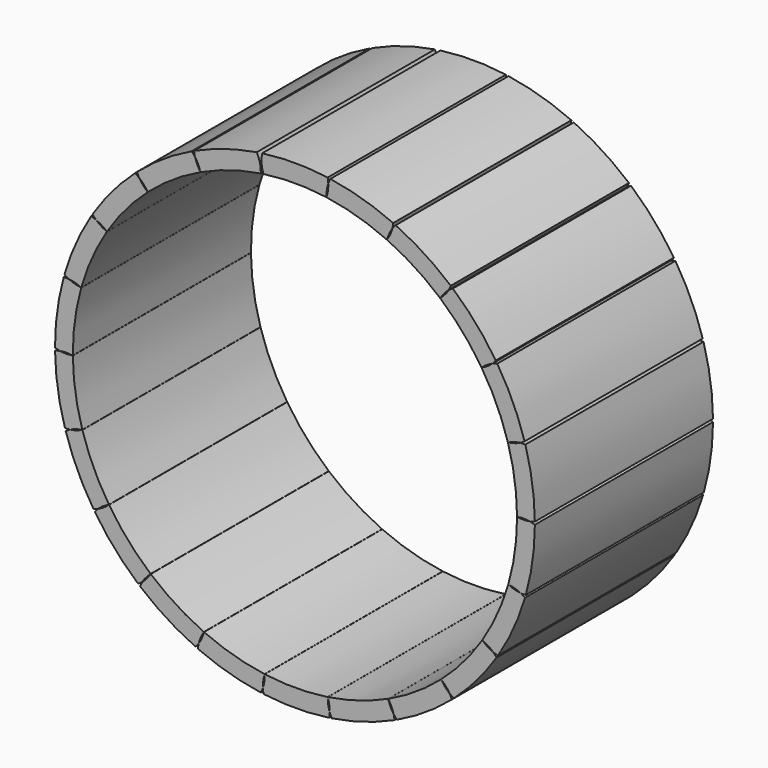
from build123d import *

# Parameters (mm, degrees)
F1_DEPTH      = 5
F1_DEPTH_BACK = 5


with BuildPart() as f1:
    # F0 (on Front) → F1 (new body, two sides)
    with BuildSketch(Plane.XZ) as f1_sk:
        with BuildLine():
            ThreePointArc((1.4985057046, 10.441937681), (1.4996263796, 10.408477179), (1.5, 10.375))
            ThreePointArc((1.5, 10.375), (1.4796631944, 10.1288357639), (1.4192042252, 9.8893464534))
            ThreePointArc((1.4192042252, 9.8893464534), (1.4195814524, 9.8813770901), (1.4200010621, 9.8734098458))
            ThreePointArc((1.4200010621, 9.8734098458), (2.8052199084, 9.5724273967), (4.1337871536, 9.0781291448))
            ThreePointArc((4.1337871536, 9.0781291448), (4.1384407168, 9.084609685), (4.1430597453, 9.0911148852))
            ThreePointArc((4.1430597453, 9.0911148852), (4.2349711699, 9.3559736019), (4.3745632608, 9.5991029871))
            ThreePointArc((4.3745632608, 9.5991029871), (4.3979930653, 9.7138757212), (4.4123952899, 9.830126795))
            ThreePointArc((4.4123952899, 9.830126795), (3.0301999512, 10.3401408721), (1.5913530114, 10.6568391464))
            ThreePointArc((1.5913530114, 10.6568391464), (1.5407305697, 10.5512024832), (1.4985057046, 10.441937681))
        make_face()
    extrude(amount=F1_DEPTH)
    extrude(f1_sk.sketch, amount=-F1_DEPTH_BACK)


with BuildPart() as f1b:
    # F0 (on Front) → F1, piece 2 (new body, two sides)
    with BuildSketch(Plane.XZ) as f1_2_sk:
        with BuildLine():
            ThreePointArc((1.4192042252, 9.8893464534), (1.4329213675, 10.1693637561), (1.4985057046, 10.441937681))
            ThreePointArc((1.4985057046, 10.441937681), (1.4887129572, 10.5586674472), (1.4698412201, 10.6742771084))
            ThreePointArc((1.4698412201, 10.6742771084), (0, 10.775), (-1.4698412201, 10.6742771084))
            ThreePointArc((-1.4698412201, 10.6742771084), (-1.496353621, 10.2704732533), (-1.4139577737, 9.8742771084))
            ThreePointArc((-1.4139577737, 9.8742771084), (0, 9.975), (1.4139577737, 9.8742771084))
            ThreePointArc((1.4139577737, 9.8742771084), (1.4166010374, 9.8818048046), (1.4192042252, 9.8893464534))
        make_face()
    extrude(amount=F1_DEPTH)
    extrude(f1_2_sk.sketch, amount=-F1_DEPTH_BACK)


with BuildPart() as f1c:
    # F0 (on Front) → F1, piece 3 (new body, two sides)
    with BuildSketch(Plane.XZ) as f1_3_sk:
        with BuildLine():
            ThreePointArc((-1.5333564365, 9.9216618431), (-1.5795383622, 10.2910031579), (-1.7152404456, 10.6376019485))
            ThreePointArc((-1.7152404456, 10.6376019485), (-3.1503051184, 10.3041837455), (-4.5264727442, 9.7781219821))
            ThreePointArc((-4.5264727442, 9.7781219821), (-4.5107188823, 9.6620463513), (-4.4859552526, 9.5475539984))
            ThreePointArc((-4.4859552526, 9.5475539984), (-4.343543736, 9.3060652622), (-4.2485568314, 9.0422938881))
            ThreePointArc((-4.2485568314, 9.0422938881), (-4.2438624259, 9.0358428719), (-4.2391337748, 9.0294169158))
            ThreePointArc((-4.2391337748, 9.0294169158), (-2.9164077546, 9.5391399407), (-1.5347846874, 9.8562194052))
            ThreePointArc((-1.5347846874, 9.8562194052), (-1.5337135417, 9.8889328324), (-1.5333564365, 9.9216618431))
        make_face()
    extrude(amount=F1_DEPTH)
    extrude(f1_3_sk.sketch, amount=-F1_DEPTH_BACK)


with BuildPart() as f1d:
    # F0 (on Front) → F1, piece 4 (new body, two sides)
    with BuildSketch(Plane.XZ) as f1_4_sk:
        with BuildLine():
            ThreePointArc((4.5240990976, 9.779220437), (4.445812008, 9.6920833735), (4.3745632608, 9.5991029871))
            ThreePointArc((4.3745632608, 9.5991029871), (4.2826518361, 9.3342442704), (4.1430597453, 9.0911148852))
            ThreePointArc((4.1430597453, 9.0911148852), (4.1411805637, 9.0833610649), (4.13934265, 9.0755973592))
            ThreePointArc((4.13934265, 9.0755973592), (5.3840128131, 8.3972037625), (6.5199524821, 7.5492280818))
            ThreePointArc((6.5199524821, 7.5492280818), (6.5262407264, 7.5541383809), (6.5325027647, 7.5590820566))
            ThreePointArc((6.5325027647, 7.5590820566), (6.6951897205, 7.7874037687), (6.8975222064, 7.9814641071))
            ThreePointArc((6.8975222064, 7.9814641071), (6.9522833955, 8.0850157773), (6.9987970873, 8.1925249057))
            ThreePointArc((6.9987970873, 8.1925249057), (5.8158133394, 9.0706637134), (4.5240990976, 9.779220437))
        make_face()
    extrude(amount=F1_DEPTH)
    extrude(f1_4_sk.sketch, amount=-F1_DEPTH_BACK)


with BuildPart() as f1e:
    # F0 (on Front) → F1, piece 5 (new body, two sides)
    with BuildSketch(Plane.XZ) as f1_5_sk:
        with BuildLine():
            ThreePointArc((-4.2485568314, 9.0422938881), (-4.390968348, 9.2837826244), (-4.4859552526, 9.5475539984))
            ThreePointArc((-4.4859552526, 9.5475539984), (-4.5582810283, 9.6396990926), (-4.6375766814, 9.7259193665))
            ThreePointArc((-4.6375766814, 9.7259193665), (-5.9209592387, 9.002381168), (-7.0936455296, 8.1105374729))
            ThreePointArc((-7.0936455296, 8.1105374729), (-7.0458840891, 8.0035768212), (-6.9899217557, 7.9006693216))
            ThreePointArc((-6.9899217557, 7.9006693216), (-6.7853450225, 7.7089763118), (-6.6200124954, 7.4825629612))
            ThreePointArc((-6.6200124954, 7.4825629612), (-6.6136933601, 7.4776924806), (-6.6073484088, 7.4728556793))
            ThreePointArc((-6.6073484088, 7.4728556793), (-5.4813520563, 8.3339909188), (-4.2446594372, 9.0268206619))
            ThreePointArc((-4.2446594372, 9.0268206619), (-4.2465875593, 9.0345624574), (-4.2485568314, 9.0422938881))
        make_face()
    extrude(amount=F1_DEPTH)
    extrude(f1_5_sk.sketch, amount=-F1_DEPTH_BACK)


with BuildPart() as f1f:
    # F0 (on Front) → F1, piece 6 (new body, two sides)
    with BuildSketch(Plane.XZ) as f1_6_sk:
        with BuildLine():
            ThreePointArc((7.091676592, 8.1122591252), (6.9920438997, 8.0506550438), (6.8975222064, 7.9814641071))
            ThreePointArc((6.8975222064, 7.9814641071), (6.7348352505, 7.753142395), (6.5325027647, 7.5590820566))
            ThreePointArc((6.5325027647, 7.5590820566), (6.5285188549, 7.5521696391), (6.5245717674, 7.5452361296))
            ThreePointArc((6.5245717674, 7.5452361296), (7.5282280627, 6.5441888142), (8.3798512956, 5.4109811739))
            ThreePointArc((8.3798512956, 5.4109811739), (8.387266657, 5.4139248905), (8.3946662565, 5.4169080066))
            ThreePointArc((8.3946662565, 5.4169080066), (8.6149972525, 5.5902634276), (8.8637386015, 5.7195908845))
            ThreePointArc((8.8637386015, 5.7195908845), (8.9454110539, 5.8035631819), (9.0202817993, 5.8936526247))
            ThreePointArc((9.0202817993, 5.8936526247), (8.1319957269, 7.0690360374), (7.091676592, 8.1122591252))
        make_face()
    extrude(amount=F1_DEPTH)
    extrude(f1_6_sk.sketch, amount=-F1_DEPTH_BACK)


with BuildPart() as f1g:
    # F0 (on Front) → F1, piece 7 (new body, two sides)
    with BuildSketch(Plane.XZ) as f1_7_sk:
        with BuildLine():
            ThreePointArc((-6.6200124954, 7.4825629612), (-6.8245892287, 7.6742559711), (-6.9899217557, 7.9006693216))
            ThreePointArc((-6.9899217557, 7.9006693216), (-7.0852421056, 7.9687557896), (-7.1855848335, 8.029196448))
            ThreePointArc((-7.1855848335, 8.029196448), (-8.2136953691, 6.9739395884), (-9.0882454133, 5.7883002953))
            ThreePointArc((-9.0882454133, 5.7883002953), (-9.0123315214, 5.6990880918), (-8.9296875575, 5.6160717593))
            ThreePointArc((-8.9296875575, 5.6160717593), (-8.679458287, 5.4896472285), (-8.4571251692, 5.318867152))
            ThreePointArc((-8.4571251692, 5.318867152), (-8.4496913613, 5.3159703342), (-8.4422422509, 5.3131130966))
            ThreePointArc((-8.4422422509, 5.3131130966), (-7.6038618382, 6.4561528905), (-6.6119209341, 7.4688102507))
            ThreePointArc((-6.6119209341, 7.4688102507), (-6.6159484275, 7.4756973655), (-6.6200124954, 7.4825629612))
        make_face()
    extrude(amount=F1_DEPTH)
    extrude(f1_7_sk.sketch, amount=-F1_DEPTH_BACK)


with BuildPart() as f1h:
    # F0 (on Front) → F1, piece 8 (new body, two sides)
    with BuildSketch(Plane.XZ) as f1_8_sk:
        with BuildLine():
            ThreePointArc((9.0868401101, 5.7905061793), (8.9739037984, 5.7594075343), (8.8637386015, 5.7195908845))
            ThreePointArc((8.8637386015, 5.7195908845), (8.6434076054, 5.5462354635), (8.3946662565, 5.4169080066))
            ThreePointArc((8.3946662565, 5.4169080066), (8.3888991849, 5.4113949367), (8.3831615181, 5.4058512707))
            ThreePointArc((8.3831615181, 5.4058512707), (9.0647925115, 4.1629510835), (9.5633594221, 2.8359798244))
            ThreePointArc((9.5633594221, 2.8359798244), (9.5713033601, 2.8367193526), (9.5792432523, 2.8375011229))
            ThreePointArc((9.5792432523, 2.8375011229), (9.8394339832, 2.9418976426), (10.1145067111, 2.9960533827))
            ThreePointArc((10.1145067111, 2.9960533827), (10.2164981278, 3.0536683733), (10.3136826364, 3.1190664429))
            ThreePointArc((10.3136826364, 3.1190664429), (9.7917934147, 4.496821847), (9.0868401101, 5.7905061793))
        make_face()
    extrude(amount=F1_DEPTH)
    extrude(f1_8_sk.sketch, amount=-F1_DEPTH_BACK)


with BuildPart() as f1i:
    # F0 (on Front) → F1, piece 9 (new body, two sides)
    with BuildSketch(Plane.XZ) as f1_9_sk:
        with BuildLine():
            ThreePointArc((-8.4571251692, 5.318867152), (-8.7073544397, 5.4452916828), (-8.9296875575, 5.6160717593))
            ThreePointArc((-8.9296875575, 5.6160717593), (-9.0403085745, 5.6546039126), (-9.1535990823, 5.6843864084))
            ThreePointArc((-9.1535990823, 5.6843864084), (-9.8434523061, 4.3825873291), (-10.3492756498, 2.9988528682))
            ThreePointArc((-10.3492756498, 2.9988528682), (-10.2513367959, 2.9345899931), (-10.1486819174, 2.8781655998))
            ThreePointArc((-10.1486819174, 2.8781655998), (-9.8729976933, 2.82721407), (-9.611609894, 2.7258520053))
            ThreePointArc((-9.611609894, 2.7258520053), (-9.6036614431, 2.7251626707), (-9.5957094382, 2.7245156224))
            ThreePointArc((-9.5957094382, 2.7245156224), (-9.11261594, 4.0571980147), (-8.4454925616, 5.3079450254))
            ThreePointArc((-8.4454925616, 5.3079450254), (-8.451294342, 5.3134215568), (-8.4571251692, 5.318867152))
        make_face()
    extrude(amount=F1_DEPTH)
    extrude(f1_9_sk.sketch, amount=-F1_DEPTH_BACK)


with BuildPart() as f1j:
    # F0 (on Front) → F1, piece 10 (new body, two sides)
    with BuildSketch(Plane.XZ) as f1_10_sk:
        with BuildLine():
            ThreePointArc((10.3485474119, 3.0013649334), (10.2314232833, 3.0032818926), (10.1145067111, 2.9960533827))
            ThreePointArc((10.1145067111, 2.9960533827), (9.8543159802, 2.8916568629), (9.5792432523, 2.8375011229))
            ThreePointArc((9.5792432523, 2.8375011229), (9.5721585158, 2.8338323953), (9.5650933928, 2.8301260372))
            ThreePointArc((9.5650933928, 2.8301260372), (9.8696803448, 1.4456952966), (9.9749484511, 0.0320686441))
            ThreePointArc((9.9749484511, 0.0320686441), (9.9827797603, 0.030544292), (9.9906190665, 0.0290616148))
            ThreePointArc((9.9906190665, 0.0290616148), (10.2696678962, 0.0560727313), (10.548869147, 0.030685503))
            ThreePointArc((10.548869147, 0.030685503), (10.6629471571, 0.0572927172), (10.7746010538, 0.0927207228))
            ThreePointArc((10.7746010538, 0.0927207228), (10.6612336557, 1.561640784), (10.3485474119, 3.0013649334))
        make_face()
    extrude(amount=F1_DEPTH)
    extrude(f1_10_sk.sketch, amount=-F1_DEPTH_BACK)


with BuildPart() as f1k:
    # F0 (on Front) → F1, piece 11 (new body, two sides)
    with BuildSketch(Plane.XZ) as f1_11_sk:
        with BuildLine():
            ThreePointArc((-9.611609894, 2.7258520053), (-9.887294118, 2.7768035352), (-10.1486819174, 2.8781655998))
            ThreePointArc((-10.1486819174, 2.8781655998), (-10.265674681, 2.8840332651), (-10.3827685769, 2.8807536652))
            ThreePointArc((-10.3827685769, 2.8807536652), (-10.6786820811, 1.4374887861), (-10.7749505298, -0.0326509008))
            ThreePointArc((-10.7749505298, -0.0326509008), (-10.6628919769, -0.0667773854), (-10.548512107, -0.0920554705))
            ThreePointArc((-10.548512107, -0.0920554705), (-10.269625143, -0.06342138), (-9.9902809211, -0.0871838608))
            ThreePointArc((-9.9902809211, -0.0871838608), (-9.9824593969, -0.0856100716), (-9.9746463541, -0.0839947032))
            ThreePointArc((-9.9746463541, -0.0839947032), (-9.8858332955, 1.3307610804), (-9.5973751813, 2.7186420562))
            ThreePointArc((-9.5973751813, 2.7186420562), (-9.6044829504, 2.7222659589), (-9.611609894, 2.7258520053))
        make_face()
    extrude(amount=F1_DEPTH)
    extrude(f1_11_sk.sketch, amount=-F1_DEPTH_BACK)


with BuildPart() as f1l:
    # F0 (on Front) → F1, piece 12 (new body, two sides)
    with BuildSketch(Plane.XZ) as f1_12_sk:
        with BuildLine():
            ThreePointArc((10.7749581379, -0.0300354193), (10.6631000201, 0.0047424144), (10.548869147, 0.030685503))
            ThreePointArc((10.548869147, 0.030685503), (10.2698203173, 0.0036743865), (9.9906190665, 0.0290616148))
            ThreePointArc((9.9906190665, 0.0290616148), (9.9827885188, 0.0275333558), (9.9749662104, 0.0259634689))
            ThreePointArc((9.9749662104, 0.0259634689), (9.9749915526, 0.0129817455), (9.975, 0))
            ThreePointArc((9.975, 0), (9.8761089107, -1.4011059144), (9.5813964344, -2.7744309988))
            ThreePointArc((9.5813964344, -2.7744309988), (9.5884830004, -2.7780961913), (9.5955889607, -2.7817236396))
            ThreePointArc((9.5955889607, -2.7817236396), (9.870972097, -2.834278164), (10.1317657755, -2.9371591972))
            ThreePointArc((10.1317657755, -2.9371591972), (10.2487224227, -2.9437073956), (10.3658334169, -2.9411090721))
            ThreePointArc((10.3658334169, -2.9411090721), (10.6701384407, -1.4995901628), (10.7749581379, -0.0300354193))
        make_face()
    extrude(amount=F1_DEPTH)
    extrude(f1_12_sk.sketch, amount=-F1_DEPTH_BACK)


with BuildPart() as f1m:
    # F0 (on Front) → F1, piece 13 (new body, two sides)
    with BuildSketch(Plane.XZ) as f1_13_sk:
        with BuildLine():
            ThreePointArc((-9.9902809211, -0.0871838608), (-10.2691678851, -0.1158179513), (-10.548512107, -0.0920554705))
            ThreePointArc((-10.548512107, -0.0920554705), (-10.6624333929, -0.1193259097), (-10.7738792894, -0.1554028881))
            ThreePointArc((-10.7738792894, -0.1554028881), (-10.6519680276, -1.6236385495), (-10.3309111471, -3.0615192096))
            ThreePointArc((-10.3309111471, -3.0615192096), (-10.2137778483, -3.0627547397), (-10.0969053081, -3.0548461629))
            ThreePointArc((-10.0969053081, -3.0548461629), (-9.8373263314, -2.9489376901), (-9.5625733222, -2.8931825672))
            ThreePointArc((-9.5625733222, -2.8931825672), (-9.5555100492, -2.8894726847), (-9.5484666084, -2.8857252863))
            ThreePointArc((-9.5484666084, -2.8857252863), (-9.861102652, -1.5030899797), (-9.9745930769, -0.0900996718))
            ThreePointArc((-9.9745930769, -0.0900996718), (-9.9824331218, -0.0886209059), (-9.9902809211, -0.0871838608))
        make_face()
    extrude(amount=F1_DEPTH)
    extrude(f1_13_sk.sketch, amount=-F1_DEPTH_BACK)


with BuildPart() as f1n:
    # F0 (on Front) → F1, piece 14 (new body, two sides)
    with BuildSketch(Plane.XZ) as f1_14_sk:
        with BuildLine():
            ThreePointArc((10.1317657755, -2.9371591972), (9.8563826392, -2.8846046729), (9.5955889607, -2.7817236396))
            ThreePointArc((9.5955889607, -2.7817236396), (9.5876446547, -2.7809880747), (9.5796965487, -2.7802947747))
            ThreePointArc((9.5796965487, -2.7802947747), (9.0888580378, -4.1101441056), (8.4144694391, -5.3569888051))
            ThreePointArc((8.4144694391, -5.3569888051), (8.4202392604, -5.3624989971), (8.4260383079, -5.3679784224))
            ThreePointArc((8.4260383079, -5.3679784224), (8.6755278398, -5.4958565803), (8.8968636424, -5.667927241))
            ThreePointArc((8.8968636424, -5.667927241), (9.0072586175, -5.7071023056), (9.1203739416, -5.7375433912))
            ThreePointArc((9.1203739416, -5.7375433912), (9.8177890082, -4.4397797231), (10.3316539871, -3.0590114237))
            ThreePointArc((10.3316539871, -3.0590114237), (10.2340906548, -2.9941798541), (10.1317657755, -2.9371591972))
        make_face()
    extrude(amount=F1_DEPTH)
    extrude(f1_14_sk.sketch, amount=-F1_DEPTH_BACK)


with BuildPart() as f1o:
    # F0 (on Front) → F1, piece 15 (new body, two sides)
    with BuildSketch(Plane.XZ) as f1_15_sk:
        with BuildLine():
            ThreePointArc((-9.5625733222, -2.8931825672), (-9.8221522989, -2.9990910401), (-10.0969053081, -3.0548461629))
            ThreePointArc((-10.0969053081, -3.0548461629), (-10.1985598103, -3.1130535371), (-10.2953622058, -3.1790158934))
            ThreePointArc((-10.2953622058, -3.1790158934), (-9.7654664053, -4.5537117703), (-9.0529987229, -5.8432729804))
            ThreePointArc((-9.0529987229, -5.8432729804), (-8.940245246, -5.8115178286), (-8.8303135559, -5.771060941))
            ThreePointArc((-8.8303135559, -5.771060941), (-8.6109948238, -5.5964266272), (-8.3630100768, -5.4656542486))
            ThreePointArc((-8.3630100768, -5.4656542486), (-8.3572751764, -5.4601077207), (-8.3515698582, -5.4545307684))
            ThreePointArc((-8.3515698582, -5.4545307684), (-9.0404201757, -4.2156171609), (-9.5466986112, -2.8915688866))
            ThreePointArc((-9.5466986112, -2.8915688866), (-9.5546381124, -2.892354618), (-9.5625733222, -2.8931825672))
        make_face()
    extrude(amount=F1_DEPTH)
    extrude(f1_15_sk.sketch, amount=-F1_DEPTH_BACK)


with BuildPart() as f1p:
    # F0 (on Front) → F1, piece 16 (new body, two sides)
    with BuildSketch(Plane.XZ) as f1_16_sk:
        with BuildLine():
            ThreePointArc((8.8968636424, -5.667927241), (8.6473741105, -5.5400490831), (8.4260383079, -5.3679784224))
            ThreePointArc((8.4260383079, -5.3679784224), (8.4186214787, -5.3650384057), (8.411189117, -5.3621378794))
            ThreePointArc((8.411189117, -5.3621378794), (7.5661729939, -6.5002808575), (6.568357508, -7.5071502347))
            ThreePointArc((6.568357508, -7.5071502347), (6.5723448659, -7.5140606638), (6.5763689229, -7.520949787))
            ThreePointArc((6.5763689229, -7.520949787), (6.7798269756, -7.7138297253), (6.9438394926, -7.9412011044))
            ThreePointArc((6.9438394926, -7.9412011044), (7.0387621206, -8.0098409684), (7.1387515229, -8.070864371))
            ThreePointArc((7.1387515229, -8.070864371), (8.1729838606, -7.0216066406), (9.0544168355, -5.8410753093))
            ThreePointArc((9.0544168355, -5.8410753093), (8.979023241, -5.751422969), (8.8968636424, -5.667927241))
        make_face()
    extrude(amount=F1_DEPTH)
    extrude(f1_16_sk.sketch, amount=-F1_DEPTH_BACK)


with BuildPart() as f1q:
    # F0 (on Front) → F1, piece 17 (new body, two sides)
    with BuildSketch(Plane.XZ) as f1_17_sk:
        with BuildLine():
            ThreePointArc((-8.3630100768, -5.4656542486), (-8.5823288088, -5.6402885624), (-8.8303135559, -5.771060941))
            ThreePointArc((-8.8303135559, -5.771060941), (-8.911496098, -5.8555069657), (-8.9858414601, -5.9460304618))
            ThreePointArc((-8.9858414601, -5.9460304618), (-8.0907323554, -7.1162261736), (-7.0443616343, -8.1533793095))
            ThreePointArc((-7.0443616343, -8.1533793095), (-6.945089024, -8.0911966345), (-6.8509714647, -8.0214569668))
            ThreePointArc((-6.8509714647, -8.0214569668), (-6.6896155764, -7.7921926497), (-6.4884155055, -7.5969584794))
            ThreePointArc((-6.4884155055, -7.5969584794), (-6.4844718777, -7.5900230015), (-6.4805651944, -7.5830666462))
            ThreePointArc((-6.4805651944, -7.5830666462), (-7.490028329, -6.5878752744), (-8.3482298473, -5.4596413267))
            ThreePointArc((-8.3482298473, -5.4596413267), (-8.3556279575, -5.4626281341), (-8.3630100768, -5.4656542486))
        make_face()
    extrude(amount=F1_DEPTH)
    extrude(f1_17_sk.sketch, amount=-F1_DEPTH_BACK)


with BuildPart() as f1r:
    # F0 (on Front) → F1, piece 18 (new body, two sides)
    with BuildSketch(Plane.XZ) as f1_18_sk:
        with BuildLine():
            ThreePointArc((6.9438394926, -7.9412011044), (6.7403814399, -7.7483211662), (6.5763689229, -7.520949787))
            ThreePointArc((6.5763689229, -7.520949787), (6.5700782296, -7.5160426258), (6.5637615249, -7.5111689932))
            ThreePointArc((6.5637615249, -7.5111689932), (5.4327743743, -8.3657389153), (4.1920719867, -9.051362188))
            ThreePointArc((4.1920719867, -9.051362188), (4.1939550364, -9.0591150699), (4.1958792958, -9.0668578264))
            ThreePointArc((4.1958792958, -9.0668578264), (4.3368834858, -9.3091709878), (4.4303342319, -9.5734905063))
            ThreePointArc((4.4303342319, -9.5734905063), (4.5021227082, -9.6660548131), (4.580915413, -9.7527349487))
            ThreePointArc((4.580915413, -9.7527349487), (5.8684856023, -9.0366753696), (7.0463405547, -8.1516691412))
            ThreePointArc((7.0463405547, -8.1516691412), (6.9992021908, -8.0444324363), (6.9438394926, -7.9412011044))
        make_face()
    extrude(amount=F1_DEPTH)
    extrude(f1_18_sk.sketch, amount=-F1_DEPTH_BACK)


with BuildPart() as f1s:
    # F0 (on Front) → F1, piece 19 (new body, two sides)
    with BuildSketch(Plane.XZ) as f1_19_sk:
        with BuildLine():
            ThreePointArc((-6.4884155055, -7.5969584794), (-6.6497713938, -7.8262227965), (-6.8509714647, -8.0214569668))
            ThreePointArc((-6.8509714647, -8.0214569668), (-6.9051292912, -8.1253254705), (-6.9510167366, -8.2331033837))
            ThreePointArc((-6.9510167366, -8.2331033837), (-5.7629442329, -9.1043450489), (-4.4671296582, -9.805374935))
            ThreePointArc((-4.4671296582, -9.805374935), (-4.3893508335, -9.7177838929), (-4.318644227, -9.624390574))
            ThreePointArc((-4.318644227, -9.624390574), (-4.2282752346, -9.3590016236), (-4.0900999675, -9.1150642436))
            ThreePointArc((-4.0900999675, -9.1150642436), (-4.0882659274, -9.1072996219), (-4.086473212, -9.0995253551))
            ThreePointArc((-4.086473212, -9.0995253551), (-5.335069023, -8.4283843956), (-6.4759227631, -7.5870316571))
            ThreePointArc((-6.4759227631, -7.5870316571), (-6.4821823342, -7.5919784564), (-6.4884155055, -7.5969584794))
        make_face()
    extrude(amount=F1_DEPTH)
    extrude(f1_19_sk.sketch, amount=-F1_DEPTH_BACK)


with BuildPart() as f1t:
    # F0 (on Front) → F1, piece 20 (new body, two sides)
    with BuildSketch(Plane.XZ) as f1_20_sk:
        with BuildLine():
            ThreePointArc((4.4303342319, -9.5734905063), (4.2893300419, -9.3311773449), (4.1958792958, -9.0668578264))
            ThreePointArc((4.1958792958, -9.0668578264), (4.1912225, -9.0603796086), (4.1865313135, -9.0539262512))
            ThreePointArc((4.1865313135, -9.0539262512), (2.8608622463, -9.5559453853), (1.4774178773, -9.864981572))
            ThreePointArc((1.4774178773, -9.864981572), (1.477044626, -9.8729511226), (1.4767137687, -9.8809225457))
            ThreePointArc((1.4767137687, -9.8809225457), (1.5392998353, -10.1243570681), (1.5603589628, -10.3748244224))
            ThreePointArc((1.5603589628, -10.3748244224), (1.5600763789, -10.4039392296), (1.5592287335, -10.433043067))
            ThreePointArc((1.5592287335, -10.433043067), (1.6020885572, -10.5420603672), (1.6533247079, -10.6474007349))
            ThreePointArc((1.6533247079, -10.6474007349), (3.0903048325, -10.3223369952), (4.4695096552, -9.8042903079))
            ThreePointArc((4.4695096552, -9.8042903079), (4.4544313568, -9.6881249898), (4.4303342319, -9.5734905063))
        make_face()
    extrude(amount=F1_DEPTH)
    extrude(f1_20_sk.sketch, amount=-F1_DEPTH_BACK)


with BuildPart() as f1u:
    # F0 (on Front) → F1, piece 21 (new body, two sides)
    with BuildSketch(Plane.XZ) as f1_21_sk:
        with BuildLine():
            ThreePointArc((-4.0900999675, -9.1150642436), (-4.1804689599, -9.380453194), (-4.318644227, -9.624390574))
            ThreePointArc((-4.318644227, -9.624390574), (-4.3414059181, -9.7392976741), (-4.3551315814, -9.8556305688))
            ThreePointArc((-4.3551315814, -9.8556305688), (-2.9699925089, -10.3575947737), (-1.5293274534, -10.6659168636))
            ThreePointArc((-1.5293274534, -10.6659168636), (-1.4793204341, -10.5599874802), (-1.437731957, -10.4504788742))
            ThreePointArc((-1.437731957, -10.4504788742), (-1.4256441122, -10.1703865077), (-1.3616466468, -9.8974356435))
            ThreePointArc((-1.3616466468, -9.8974356435), (-1.3620702313, -9.8894686096), (-1.3625361852, -9.8815039414))
            ThreePointArc((-1.3625361852, -9.8815039414), (-2.7494826243, -9.588585417), (-4.0809030803, -9.1020247774))
            ThreePointArc((-4.0809030803, -9.1020247774), (-4.0855188628, -9.1085322812), (-4.0900999675, -9.1150642436))
        make_face()
    extrude(amount=F1_DEPTH)
    extrude(f1_21_sk.sketch, amount=-F1_DEPTH_BACK)


with BuildPart() as f1v:
    # F0 (on Front) → F1, piece 22 (new body, two sides)
    with BuildSketch(Plane.XZ) as f1_22_sk:
        with BuildLine():
            ThreePointArc((1.5592287335, -10.433043067), (1.4920597443, -10.160855307), (1.4767137687, -9.8809225457))
            ThreePointArc((1.4767137687, -9.8809225457), (1.4740667498, -9.8733961692), (1.4713797367, -9.8658839782))
            ThreePointArc((1.4713797367, -9.8658839782), (0.0580318703, -9.9748311917), (-1.3564879536, -9.8823360311))
            ThreePointArc((-1.3564879536, -9.8823360311), (-1.3590873784, -9.8898789777), (-1.3616466468, -9.8974356435))
            ThreePointArc((-1.3616466468, -9.8974356435), (-1.3602149126, -9.9352508278), (-1.3597375666, -9.9730900954))
            ThreePointArc((-1.3597375666, -9.9730900954), (-1.3793645706, -10.2149491303), (-1.437731957, -10.4504788742))
            ThreePointArc((-1.437731957, -10.4504788742), (-1.4272602728, -10.5671496934), (-1.4077162692, -10.6826476075))
            ThreePointArc((-1.4077162692, -10.6826476075), (0.0626860554, -10.7748176531), (1.5319164224, -10.6655453248))
            ThreePointArc((1.5319164224, -10.6655453248), (1.5501152541, -10.5498278293), (1.5592287335, -10.433043067))
        make_face()
    extrude(amount=F1_DEPTH)
    extrude(f1_22_sk.sketch, amount=-F1_DEPTH_BACK)


solid = Compound([f1.part, f1b.part, f1c.part, f1d.part, f1e.part, f1f.part, f1g.part, f1h.part, f1i.part, f1j.part, f1k.part, f1l.part, f1m.part, f1n.part, f1o.part, f1p.part, f1q.part, f1r.part, f1s.part, f1t.part, f1u.part, f1v.part])
